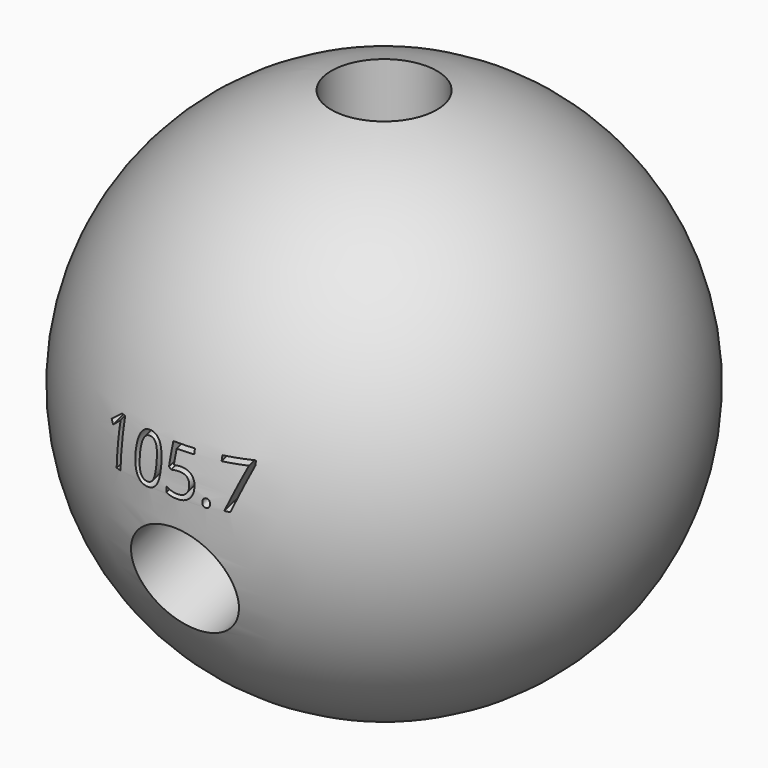
from build123d import *

# Parameters (mm, degrees)
F4_R         = 3.175
F5_DEPTH     = 50.8
F7_ANGLE     = 105.7
F9_TEXT_SIZE = 3.5808680372
F10_DEPTH    = 20.1422


# Not quite as in the source:
# - Text() gives the source's letters only with a copy of the font that has no kerning and outlines rounded to 1/6400 em; it was checked with that copy


with BuildPart() as f2:
    # F0 (on Front) → F2 (revolve)
    with BuildSketch(Plane.XZ):
        with BuildLine():
            Line((0, -15.875), (0, 15.875))
            ThreePointArc((0, 15.875), (-15.875, 0), (0, -15.875))
        make_face()
    revolve(axis=Axis((0, 0, 0), (0, 0, 1)))

    # F9 (on offset) → F10 (cut)
    with BuildSketch(Plane(origin=(0, -30.565462949, -8.5915641597), x_dir=(1, 0, 0), z_dir=(0, -0.9626917464, -0.270600446))):
        with Locations((-4.7258026898, 4.7506955452)):
            Text('105.7', F9_TEXT_SIZE, font='Open Sans', text_align=(TextAlign.LEFT, TextAlign.BOTTOM))
    extrude(amount=-F10_DEPTH, mode=Mode.SUBTRACT)


with BuildPart() as f5:
    # F4 (on offset) → F5 (new body)
    with BuildSketch(Plane.XY.offset(6.35)):
        Circle(F4_R)
    extrude(amount=F5_DEPTH)


with BuildPart() as f7_1:
    # F7: copy of F5
    add(f5.part.rotate(Axis((33.4546864033, 0, 0), (1, 0, 0)), F7_ANGLE))


with BuildPart() as f2_1:
    add(f2.part)

    # F11: cut F5, F7_1
    add(f5.part, mode=Mode.SUBTRACT)
    add(f7_1.part, mode=Mode.SUBTRACT)


solid = f2_1.part
